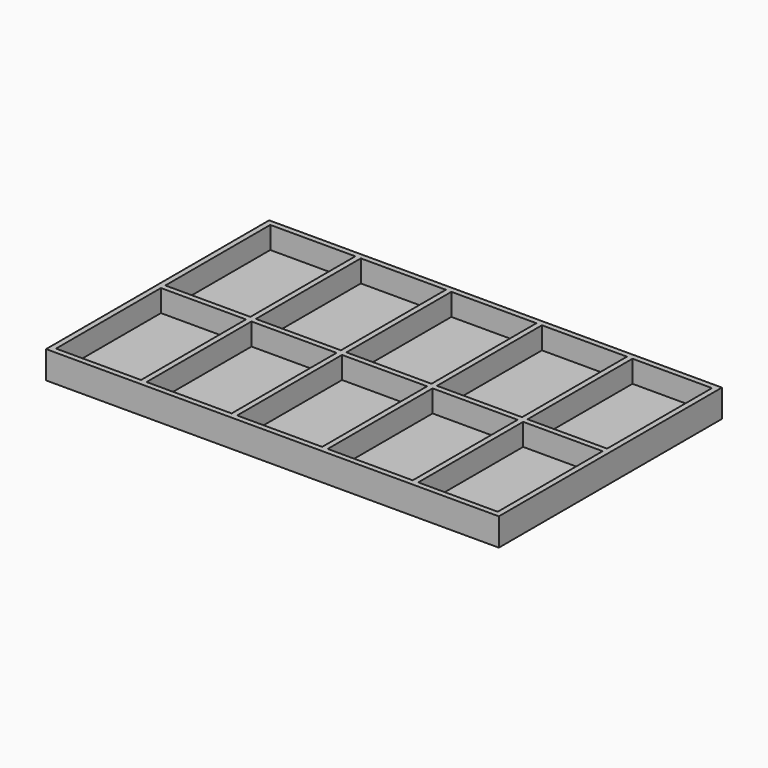
from build123d import *

# Parameters (mm, degrees)
F0_W     = 164
F0_H     = 101
F1_DEPTH = 10
F2_W     = 160
F2_H     = 97
F3_DEPTH = 8
F4_W     = 160
F4_H     = 2
F5_DEPTH = 8
F6_W     = 2
F6_H     = 97
F7_DEPTH = 8
F8_R     = 5
F9_DEPTH = 1
F10_SIZE = 0.99999


# Not quite as in the source:
# - a fillet or chamfer is up to 0.001 mm smaller than in the source, because OpenCascade refuses the exact size


with BuildPart() as f1:
    # F0 (on Top) → F1 (new body)
    with BuildSketch(Plane.XY):
        Rectangle(F0_W, F0_H)
    extrude(amount=F1_DEPTH)

    # F2 (on face) → F3 (cut)
    with BuildSketch(Plane.XY.offset(10)):
        Rectangle(F2_W, F2_H)
    extrude(amount=-F3_DEPTH, mode=Mode.SUBTRACT)

    # F4 (on face) → F5 (join)
    with BuildSketch(Plane.XY.offset(2)):
        Rectangle(F4_W, F4_H)
    extrude(amount=F5_DEPTH)

    # F6 (on face) → F7 (join)
    with BuildSketch(Plane.XY.offset(2)):
        with Locations((-48.2, 0)):
            Rectangle(F6_W, F6_H)
        with Locations((-15.4, 0)):
            Rectangle(F6_W, F6_H)
        with Locations((17.4, 0)):
            Rectangle(F6_W, F6_H)
        with Locations((50.2, 0)):
            Rectangle(F6_W, F6_H)
    extrude(amount=F7_DEPTH)

    # F8 (on face) → F9 (join)
    with BuildSketch(Plane(origin=(0, 0, 0), x_dir=(1, 0, 0), z_dir=(0, 0, -1))):
        with Locations((-67, 35.5)):
            Circle(F8_R)
        with Locations((67, 35.5)):
            Circle(F8_R)
        with Locations((67, -35.5)):
            Circle(F8_R)
        with Locations((-67, -35.5)):
            Circle(F8_R)
    extrude(amount=F9_DEPTH)

    # F10 (size 1 in the source; OpenCascade refuses exactly that, so slightly less here)
    f10_edges = [f1.edges().sort_by_distance(p)[0] for p in [
        (-72, -35.5, -1),
        (-72, 35.5, -1),
        (62, -35.5, -1),
        (62, 35.5, -1),
    ]]
    chamfer(f10_edges, length=F10_SIZE)


solid = f1.part
